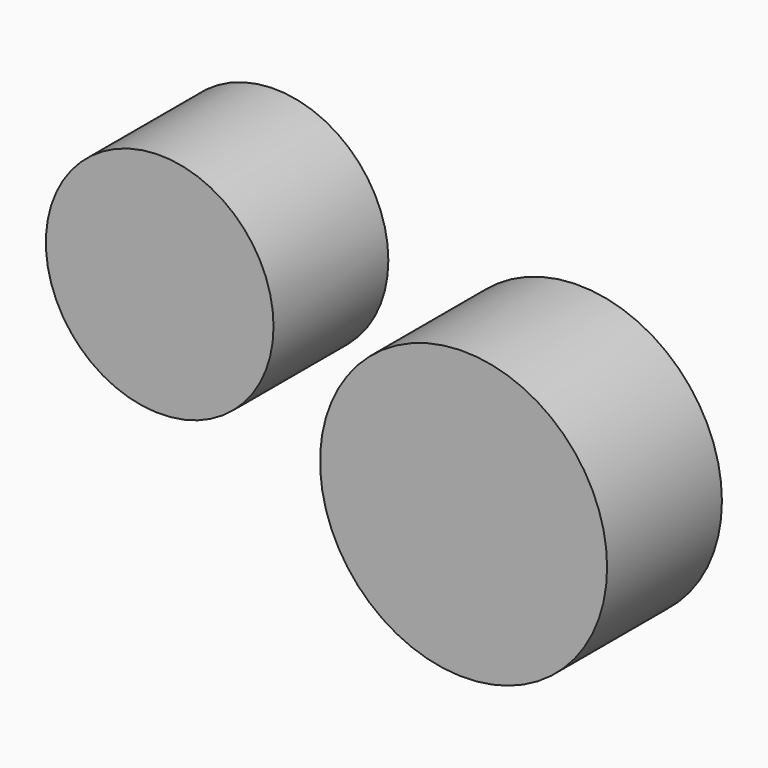
from build123d import *

# Parameters (mm, degrees)
F0_R     = 76.2
F1_DEPTH = 76.2
F0_R_2   = 60.4382074191


# Not quite as in the source:
# - the program builds the solid bodies; features that only make, move or delete a surface that nothing else refers to are left out


with BuildPart() as f1:
    # F0 (on Front) → F1 (new body)
    with BuildSketch(Plane.XZ):
        with Locations((70.2530217951, -40.6267557943)):
            Circle(F0_R)
    extrude(amount=F1_DEPTH)


with BuildPart() as f1b:
    # F0 (on Front) → F1, piece 2 (new body)
    with BuildSketch(Plane.XZ):
        with Locations((-91.0844604408, 14.3582018072)):
            Circle(F0_R_2)
    extrude(amount=F1_DEPTH)


solid = Compound([f1.part, f1b.part])
